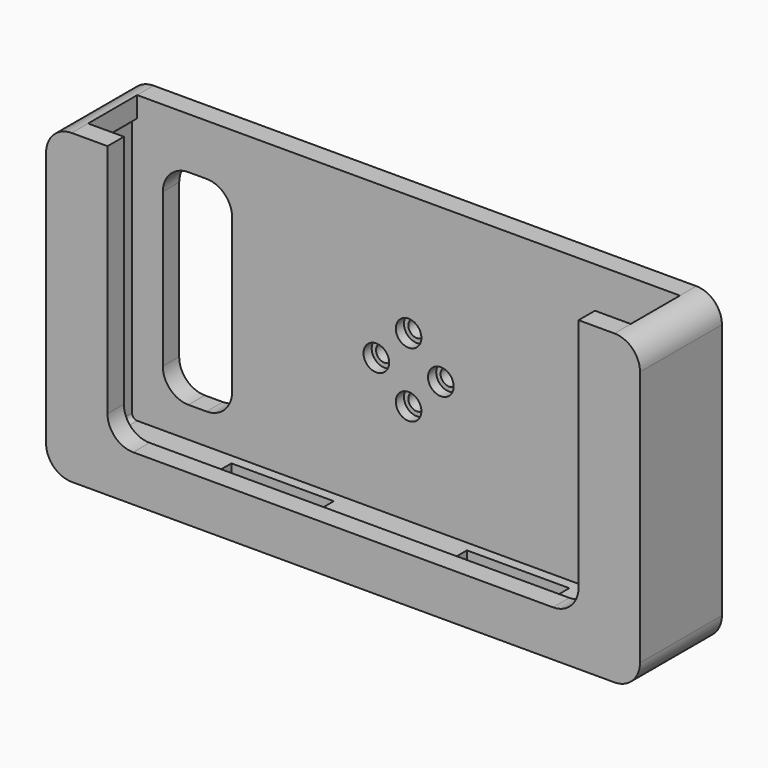
from build123d import *

# Parameters (mm, degrees)
F1_DEPTH  = 25.4
F2_T      = -5.08
F4_DEPTH  = 5.08
F6_DEPTH  = 5.08
F7_R      = 2.0955
F8_DEPTH  = 5.08
F9_R      = 3.175
F9_R_2    = 2.0955
F10_DEPTH = 2.54
F11_W     = 25.4
F11_H     = 12.7
F12_DEPTH = 5.08


# Not quite as in the source:
# - a shell that OpenCascade refuses in one call is made with other operations: the cavity is built on its own and cut out


with BuildPart() as f1:
    # F0 (on Front) → F1 (new body)
    with BuildSketch(Plane.XZ):
        with BuildLine():
            Line((43.9080937201, 75.5717812867), (-90.7119062799, 75.5717812867))
            ThreePointArc((-90.7119062799, 75.5717812867), (-95.2020343405, 73.7119093473), (-97.0619062799, 69.2217812867))
            Line((-97.0619062799, 69.2217812867), (-97.0619062799, 5.7217812867))
            ThreePointArc((-97.0619062799, 5.7217812867), (-95.2020343405, 1.2316532262), (-90.7119062799, -0.6282187133))
            Line((-90.7119062799, -0.6282187133), (43.9080937201, -0.6282187133))
            ThreePointArc((43.9080937201, -0.6282187133), (48.3982217806, 1.2316532262), (50.2580937201, 5.7217812867))
            Line((50.2580937201, 5.7217812867), (50.2580937201, 69.2217812867))
            ThreePointArc((50.2580937201, 69.2217812867), (48.3982217806, 73.7119093473), (43.9080937201, 75.5717812867))
        make_face()
    extrude(amount=F1_DEPTH)

    # F2: a shell. OpenCascade refuses it in one call, so the cavity is built on its own and cut out:
    # the body offset inwards by the wall thickness, plus a prism from it out through each open face.
    f2_core = offset(f1.part, amount=F2_T, mode=Mode.PRIVATE)
    f2_exits = [f2_core.faces().sort_by_distance(p)[0] for p in [
        (-23.401906, -12.7, 70.491781),
    ]]
    add(f2_core, mode=Mode.SUBTRACT)
    extrude(f2_exits, amount=-F2_T, mode=Mode.SUBTRACT)

    # F3 (on face) → F4 (cut)
    with BuildSketch(Plane.XZ.offset(25.4)):
        with BuildLine():
            Line((35.0180937201, 75.5717812867), (-81.8219062799, 75.5717812867))
            Line((-81.8219062799, 75.5717812867), (-81.8219062799, 17.1517812867))
            ThreePointArc((-81.8219062799, 17.1517812867), (-79.9620343405, 12.6616532262), (-75.4719062799, 10.8017812867))
            Line((-75.4719062799, 10.8017812867), (28.6680937201, 10.8017812867))
            ThreePointArc((28.6680937201, 10.8017812867), (33.1582217806, 12.6616532262), (35.0180937201, 17.1517812867))
            Line((35.0180937201, 17.1517812867), (35.0180937201, 75.5717812867))
        make_face()
    extrude(amount=-F4_DEPTH, mode=Mode.SUBTRACT)

    # F5 (on face) → F6 (cut)
    with BuildSketch(Plane(origin=(0, 0, 0), x_dir=(-1, 0, 0), z_dir=(0, 1, 0))):
        with BuildLine():
            Line((-26.1280937201, 62.8717812867), (-31.2080937201, 62.8717812867))
            ThreePointArc((-31.2080937201, 62.8717812867), (-35.6982217806, 61.0119093473), (-37.5580937201, 56.5217812867))
            Line((-37.5580937201, 56.5217812867), (-37.5580937201, 18.4217812867))
            ThreePointArc((-37.5580937201, 18.4217812867), (-35.6982217806, 13.9316532262), (-31.2080937201, 12.0717812867))
            Line((-31.2080937201, 12.0717812867), (-26.1280937201, 12.0717812867))
            ThreePointArc((-26.1280937201, 12.0717812867), (-21.6379656595, 13.9316532262), (-19.7780937201, 18.4217812867))
            Line((-19.7780937201, 18.4217812867), (-19.7780937201, 56.5217812867))
            ThreePointArc((-19.7780937201, 56.5217812867), (-21.6379656595, 61.0119093473), (-26.1280937201, 62.8717812867))
        make_face()
        with BuildLine():
            Line((78.0119062799, 62.8717812867), (73.519602201, 62.8717812867))
            ThreePointArc((73.519602201, 62.8717812867), (69.0294741405, 61.0119093473), (67.169602201, 56.5217812867))
            Line((67.169602201, 56.5217812867), (67.169602201, 18.4217812867))
            ThreePointArc((67.169602201, 18.4217812867), (69.0294741405, 13.9316532262), (73.519602201, 12.0717812867))
            Line((73.519602201, 12.0717812867), (78.0119062799, 12.0717812867))
            ThreePointArc((78.0119062799, 12.0717812867), (82.5020343405, 13.9316532262), (84.3619062799, 18.4217812867))
            Line((84.3619062799, 18.4217812867), (84.3619062799, 56.5217812867))
            ThreePointArc((84.3619062799, 56.5217812867), (82.5020343405, 61.0119093473), (78.0119062799, 62.8717812867))
        make_face()
    extrude(amount=-F6_DEPTH, mode=Mode.SUBTRACT)

    # F7 (on face) → F8 (cut)
    with BuildSketch(Plane.XZ.offset(5.08)):
        with Locations((-23.4019062799, 45.4727812867)):
            Circle(F7_R)
        with Locations((-31.4029062799, 37.4717812867)):
            Circle(F7_R)
        with Locations((-23.4019062799, 29.4707812867)):
            Circle(F7_R)
        with Locations((-15.4009062799, 37.4717812867)):
            Circle(F7_R)
    extrude(amount=-F8_DEPTH, mode=Mode.SUBTRACT)

    # F9 (on face) → F10 (cut)
    with BuildSketch(Plane.XZ.offset(5.08)):
        with Locations((-31.4029062799, 37.4717812867)):
            Circle(F9_R)
        with Locations((-31.4029062799, 37.4717812867)):
            Circle(F9_R_2, mode=Mode.SUBTRACT)
        with Locations((-23.4019062799, 45.4727812867)):
            Circle(F9_R)
        with Locations((-23.4019062799, 45.4727812867)):
            Circle(F9_R_2, mode=Mode.SUBTRACT)
        with Locations((-15.4009062799, 37.4717812867)):
            Circle(F9_R)
        with Locations((-15.4009062799, 37.4717812867)):
            Circle(F9_R_2, mode=Mode.SUBTRACT)
        with Locations((-23.4019062799, 29.4707812867)):
            Circle(F9_R)
        with Locations((-23.4019062799, 29.4707812867)):
            Circle(F9_R_2, mode=Mode.SUBTRACT)
    extrude(amount=-F10_DEPTH, mode=Mode.SUBTRACT)

    # F11 (on face) → F12 (cut)
    with BuildSketch(Plane(origin=(0, 0, -0.6282187133), x_dir=(1, 0, 0), z_dir=(0, 0, -1))):
        with Locations((-52.6119062799, 13.97)):
            Rectangle(F11_W, F11_H)
        with Locations((5.8080937201, 13.97)):
            Rectangle(F11_W, F11_H)
    extrude(amount=-F12_DEPTH, mode=Mode.SUBTRACT)


solid = f1.part
